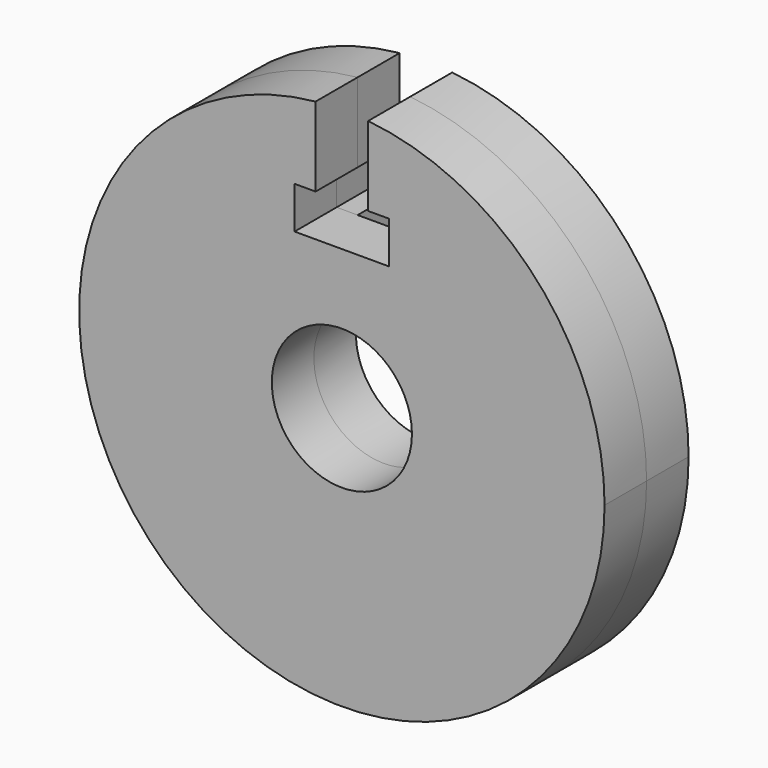
from build123d import *

# Parameters (mm, degrees)
F1_DEPTH = 3
F3_DEPTH = 3
F4_DEPTH = 25


with BuildPart() as f1:
    # F0 (on Front) → F1 (new body)
    with BuildSketch(Plane.XZ):
        with BuildLine():
            ThreePointArc((-1.5, 14.9248115566), (-10.0623058987, -11.1242977306), (15, 0))
            ThreePointArc((15, 0), (11.1242977306, 10.0623058987), (1.5, 14.9248115566))
            Line((1.5, 14.9248115566), (1.5, 10.4))
            Line((1.5, 10.4), (2.7, 10.4))
            Line((2.7, 10.4), (2.7, 8))
            Line((2.7, 8), (1.5, 8))
            Line((1.5, 8), (1.5, 3.7080992435))
            ThreePointArc((1.5, 3.7080992435), (3.3166247904, 2.2360679775), (4, 0))
            ThreePointArc((4, 0), (-2.2360679775, -3.3166247904), (-1.5, 3.7080992435))
            Line((-1.5, 3.7080992435), (-1.5, 8))
            Line((-1.5, 8), (-2.7, 8))
            Line((-2.7, 8), (-2.7, 10.4))
            Line((-2.7, 10.4), (-1.5, 10.4))
            Line((-1.5, 10.4), (-1.5, 14.9248115566))
        make_face()
    extrude(amount=F1_DEPTH)


with BuildPart() as f3:
    # F2 (on face) → F3 (new body)
    with BuildSketch(Plane.XZ.offset(3)):
        with BuildLine():
            ThreePointArc((-2.7, 9.6286032217), (-6.0415229868, -7.9686887253), (10, 0))
            ThreePointArc((10, 0), (7.9686887253, 6.0415229868), (2.7, 9.6286032217))
            Line((2.7, 9.6286032217), (2.7, 8))
            Line((2.7, 8), (1.5, 8))
            Line((1.5, 8), (1.5, 3.7080992435))
            ThreePointArc((1.5, 3.7080992435), (3.3166247904, 2.2360679775), (4, 0))
            ThreePointArc((4, 0), (-2.2360679775, -3.3166247904), (-1.5, 3.7080992435))
            Line((-1.5, 3.7080992435), (-1.5, 8))
            Line((-1.5, 8), (-2.7, 8))
            Line((-2.7, 8), (-2.7, 9.6286032217))
        make_face()
        with BuildLine():
            ThreePointArc((2.7, 9.6286032217), (7.9686887253, 6.0415229868), (10, 0))
            ThreePointArc((10, 0), (-6.0415229868, -7.9686887253), (-2.7, 9.6286032217))
            Line((-2.7, 9.6286032217), (-2.7, 10.4))
            Line((-2.7, 10.4), (-1.5, 10.4))
            Line((-1.5, 10.4), (-1.5, 14.9248115566))
            ThreePointArc((-1.5, 14.9248115566), (-10.0623058987, -11.1242977306), (15, 0))
            ThreePointArc((15, 0), (11.1242977306, 10.0623058987), (1.5, 14.9248115566))
            Line((1.5, 14.9248115566), (1.5, 10.4))
            Line((1.5, 10.4), (2.7, 10.4))
            Line((2.7, 10.4), (2.7, 9.6286032217))
        make_face()
        with BuildLine():
            Line((1.5, 3.7080992435), (1.5, 8))
            Line((1.5, 8), (-1.5, 8))
            Line((-1.5, 8), (-1.5, 3.7080992435))
            ThreePointArc((-1.5, 3.7080992435), (0, 4), (1.5, 3.7080992435))
        make_face()
        with BuildLine():
            ThreePointArc((4, 0), (3.3166247904, 2.2360679775), (1.5, 3.7080992435))
            ThreePointArc((1.5, 3.7080992435), (0, 4), (-1.5, 3.7080992435))
            ThreePointArc((-1.5, 3.7080992435), (-2.2360679775, -3.3166247904), (4, 0))
        make_face()
    extrude(amount=F3_DEPTH)

    # F2 (on face) → F4 (cut)
    with BuildSketch(Plane.XZ.offset(3)):
        with BuildLine():
            ThreePointArc((4, 0), (3.3166247904, 2.2360679775), (1.5, 3.7080992435))
            ThreePointArc((1.5, 3.7080992435), (0, 4), (-1.5, 3.7080992435))
            ThreePointArc((-1.5, 3.7080992435), (-2.2360679775, -3.3166247904), (4, 0))
        make_face()
    extrude(amount=F4_DEPTH, mode=Mode.SUBTRACT)


solid = Compound([f1.part, f3.part])
